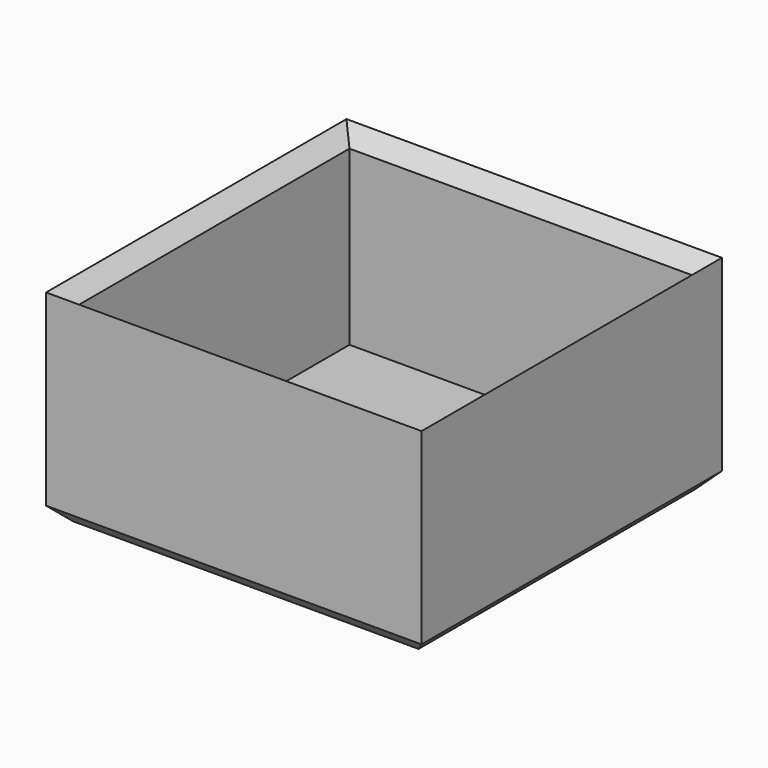
from build123d import *

# Parameters (mm, degrees)
F0_W     = 50
F0_H     = 50
F0_W_2   = 46
F0_H_2   = 46
F1_DEPTH = 25
F2_DEPTH = 2
F3_SIZE  = 1.99999


# Not quite as in the source:
# - a fillet or chamfer is up to 0.001 mm smaller than in the source, because OpenCascade refuses the exact size


with BuildPart() as f1:
    # F0 (on Top) → F1 (new body)
    with BuildSketch(Plane.XY):
        Rectangle(F0_W, F0_H)
        Rectangle(F0_W_2, F0_H_2, mode=Mode.SUBTRACT)
    extrude(amount=F1_DEPTH)

    # F0 (on Top) → F2 (join)
    with BuildSketch(Plane.XY):
        Rectangle(F0_W, F0_H)
        Rectangle(F0_W_2, F0_H_2, mode=Mode.SUBTRACT)
        Rectangle(F0_W_2, F0_H_2)
    extrude(amount=-F2_DEPTH)

    # F3 (size 2 in the source; OpenCascade refuses exactly that, so slightly less here)
    f3_edges = [f1.edges().sort_by_distance(p)[0] for p in [
        (0, -25, -2),
        (-25, 0, -2),
        (25, 0, -2),
        (0, 25, -2),
        (-23, 0, 25),
        (0, 23, 25),
        (23, 0, 25),
        (0, -23, 25),
    ]]
    chamfer(f3_edges, length=F3_SIZE)


solid = f1.part
